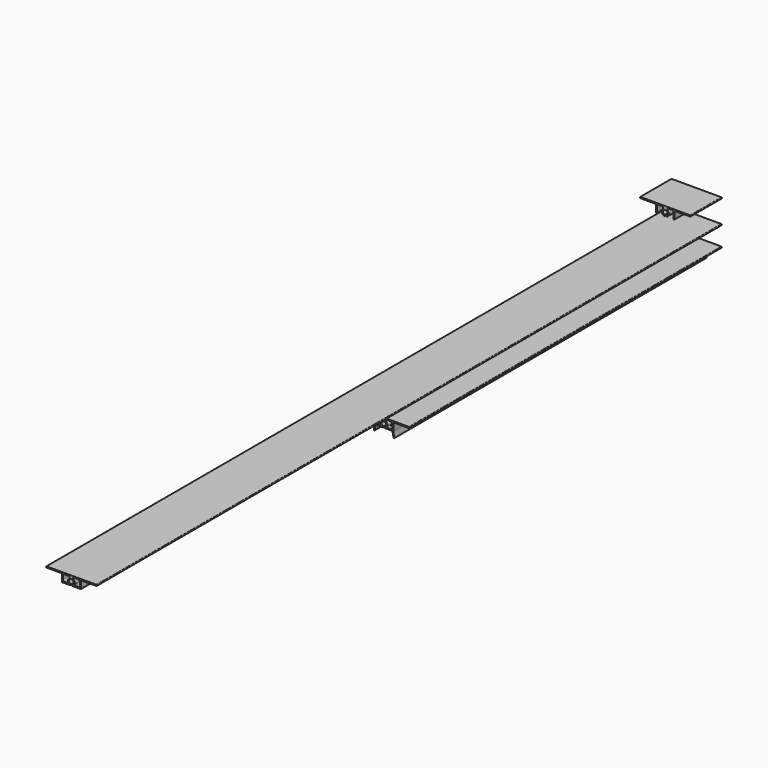
from build123d import *

# Parameters (mm, degrees)
F1_DEPTH = 1000
F2_DEPTH = 2000
F3_DEPTH = 100


# Not quite as in the source:
# - ends of sketch curves that miss each other by under 0.0002 mm in the source are joined


with BuildPart() as f1:
    # F0 (on Front) → F1 (new body)
    with BuildSketch(Plane.XZ):
        with BuildLine():
            Line((63.5, 0), (-63.5, 0))
            ThreePointArc((-63.5, 0), (-65, -1.5), (-63.5, -3))
            Line((-63.5, -3), (-25.2083473523, -3))
            ThreePointArc((-25.2083473523, -3), (-24.5012405711, -3.2928932188), (-24.2083473523, -4))
            Line((-24.2083473523, -4), (-24.2083473523, -22.8776747597))
            ThreePointArc((-24.2083473523, -22.8776747597), (-24.2120777554, -22.9997718388), (-24.223255049, -23.1214134465))
            Line((-24.223255049, -23.1214134465), (-26.0512952001, -38.0096057211))
            ThreePointArc((-26.0512952001, -38.0096057211), (-24.9164089173, -37.5089670967), (-24.2949814984, -36.4354523693))
            Line((-24.2949814984, -36.4354523693), (-21.7759150734, -24.5841766184))
            ThreePointArc((-21.7759150734, -24.5841766184), (-21.0782606541, -23.4457080771), (-19.819619872, -23))
            Line((-19.819619872, -23), (-2.7222222222, -23))
            ThreePointArc((-2.7222222222, -23), (-2.015115441, -22.7071067812), (-1.7222222222, -22))
            Line((-1.7222222222, -22), (-1.7222222222, -20.8607207227))
            ThreePointArc((-1.7222222222, -20.8607207227), (-1.8888888889, -20.3079499243), (-2.3333333333, -19.9394360587))
            ThreePointArc((-2.3333333333, -19.9394360587), (0, -8.4117280748), (2.3333333333, -19.9394360587))
            ThreePointArc((2.3333333333, -19.9394360587), (1.8888888889, -20.3079499243), (1.7222222222, -20.8607207227))
            Line((1.7222222222, -20.8607207227), (1.7222222222, -22))
            ThreePointArc((1.7222222222, -22), (2.015115441, -22.7071067812), (2.7222222222, -23))
            Line((2.7222222222, -23), (19.819619872, -23))
            ThreePointArc((19.819619872, -23), (21.0782606541, -23.4457080771), (21.7759150734, -24.5841766184))
            Line((21.7759150734, -24.5841766184), (24.2949814984, -36.4354523693))
            ThreePointArc((24.2949814984, -36.4354523693), (24.9164089173, -37.5089670967), (26.0512952001, -38.0096057211))
            Line((26.0512952001, -38.0096057211), (24.2381627457, -23.242826893))
            ThreePointArc((24.2381627457, -23.242826893), (24.2269854521, -23.1211852853), (24.223255049, -22.9990882062))
            Line((24.223255049, -22.9990882062), (24.223255049, -3))
            Line((24.223255049, -3), (63.5, -3))
            ThreePointArc((63.5, -3), (65, -1.5), (63.5, 0))
        make_face()
        with BuildLine():
            Line((-21.2083473523, -16), (-21.2083473523, -7))
            ThreePointArc((-21.2083473523, -7), (-20.036774477, -4.1715728753), (-17.2083473523, -3))
            Line((-17.2083473523, -3), (-5.6938014232, -3))
            ThreePointArc((-5.6938014232, -3), (-3.7673478716, -4.4626205124), (-4.6585648008, -6.7112232863))
            ThreePointArc((-4.6585648008, -6.7112232863), (-8.4473321852, -11.3064778509), (-8.5368852816, -17.2615683665))
            ThreePointArc((-8.5368852816, -17.2615683665), (-8.8221800029, -19.1358853065), (-10.5097115925, -20))
            Line((-10.5097115925, -20), (-17.2083473523, -20))
            ThreePointArc((-17.2083473523, -20), (-20.036774477, -18.8284271247), (-21.2083473523, -16))
        make_face(mode=Mode.SUBTRACT)
        with BuildLine():
            Line((21.2083473523, -7), (21.2083473523, -7.008646884))
            Line((21.2083473523, -7.008646884), (21.2083473523, -16))
            ThreePointArc((21.2083473523, -16), (20.036774477, -18.8284271247), (17.2083473523, -20))
            Line((17.2083473523, -20), (10.5097115925, -20))
            ThreePointArc((10.5097115925, -20), (8.8221800029, -19.1358853065), (8.5368852816, -17.2615683665))
            ThreePointArc((8.5368852816, -17.2615683665), (8.4473321852, -11.3064778509), (4.6585648008, -6.7112232863))
            ThreePointArc((4.6585648008, -6.7112232863), (3.7673478716, -4.4626205124), (5.6938014232, -3))
            Line((5.6938014232, -3), (17.2083473523, -3))
            ThreePointArc((17.2083473523, -3), (20.036774477, -4.1715728753), (21.2083473523, -7))
        make_face(mode=Mode.SUBTRACT)
    extrude(amount=F1_DEPTH)


with BuildPart() as f2:
    # F0 (on Front) → F2 (new body)
    with BuildSketch(Plane.XZ):
        with BuildLine():
            Line((63.4000037313, 50.7132201195), (-63.5999962687, 50.7132201195))
            ThreePointArc((-63.5999962687, 50.7132201195), (-65.0999962687, 49.2132201195), (-63.5999962687, 47.7132201195))
            Line((-63.5999962687, 47.7132201195), (-25.308343621, 47.7132201195))
            ThreePointArc((-25.308343621, 47.7132201195), (-24.6012368398, 47.4203269007), (-24.308343621, 46.7132201195))
            Line((-24.308343621, 46.7132201195), (-24.308343621, 28.7132201195))
            ThreePointArc((-24.308343621, 28.7132201195), (-24.0154504022, 28.0061133383), (-23.308343621, 27.7132201195))
            Line((-23.308343621, 27.7132201195), (-19.9187639256, 27.7132201195))
            Line((-19.9187639256, 27.7132201195), (-2.822218491, 27.7132201195))
            ThreePointArc((-2.822218491, 27.7132201195), (-2.1151117098, 28.0061133383), (-1.822218491, 28.7132201195))
            Line((-1.822218491, 28.7132201195), (-1.822218491, 29.8524993968))
            ThreePointArc((-1.822218491, 29.8524993968), (-1.9888851576, 30.4052701952), (-2.4333296021, 30.7737840608))
            ThreePointArc((-2.4333296021, 30.7737840608), (-0.0999962687, 42.3014920447), (2.2333370646, 30.7737840608))
            ThreePointArc((2.2333370646, 30.7737840608), (1.7888926201, 30.4052701952), (1.6222259535, 29.8524993968))
            Line((1.6222259535, 29.8524993968), (1.6222259535, 28.7132201195))
            ThreePointArc((1.6222259535, 28.7132201195), (1.9151191723, 28.0061133383), (2.6222259535, 27.7132201195))
            Line((2.6222259535, 27.7132201195), (19.7196236032, 27.7132201195))
            Line((19.7196236032, 27.7132201195), (23.629926187, 27.7132201195))
            ThreePointArc((23.629926187, 27.7132201195), (24.3370329682, 28.0061133383), (24.629926187, 28.7132201195))
            Line((24.629926187, 28.7132201195), (24.629926187, 47.7132201195))
            Line((24.629926187, 47.7132201195), (63.4000037313, 47.7132201195))
            ThreePointArc((63.4000037313, 47.7132201195), (64.9000037313, 49.2132201195), (63.4000037313, 50.7132201195))
        make_face()
        with BuildLine():
            Line((-21.308343621, 34.7132201195), (-21.308343621, 43.7132201195))
            ThreePointArc((-21.308343621, 43.7132201195), (-20.1367707458, 46.5416472442), (-17.308343621, 47.7132201195))
            Line((-17.308343621, 47.7132201195), (-5.7937976919, 47.7132201195))
            ThreePointArc((-5.7937976919, 47.7132201195), (-3.8673441404, 46.2505996071), (-4.7585610695, 44.0019968332))
            ThreePointArc((-4.7585610695, 44.0019968332), (-8.5473284539, 39.4067422686), (-8.6368815504, 33.451651753))
            ThreePointArc((-8.6368815504, 33.451651753), (-8.9221762716, 31.577334813), (-10.6097078613, 30.7132201195))
            Line((-10.6097078613, 30.7132201195), (-17.308343621, 30.7132201195))
            ThreePointArc((-17.308343621, 30.7132201195), (-20.1367707458, 31.8847929947), (-21.308343621, 34.7132201195))
        make_face(mode=Mode.SUBTRACT)
        with BuildLine():
            Line((21.629926187, 43.7218670034), (21.629926187, 43.7132201195))
            Line((21.629926187, 43.7132201195), (21.629926187, 34.7132201195))
            ThreePointArc((21.629926187, 34.7132201195), (20.4583533118, 31.8847929947), (17.629926187, 30.7132201195))
            Line((17.629926187, 30.7132201195), (17.1083510835, 30.7132201195))
            Line((17.1083510835, 30.7132201195), (10.4097153238, 30.7132201195))
            ThreePointArc((10.4097153238, 30.7132201195), (8.7221837341, 31.577334813), (8.4368890129, 33.451651753))
            ThreePointArc((8.4368890129, 33.451651753), (8.3473359164, 39.4067422686), (4.558568532, 44.0019968332))
            ThreePointArc((4.558568532, 44.0019968332), (3.6673516029, 46.2505996071), (5.5938051544, 47.7132201195))
            Line((5.5938051544, 47.7132201195), (6.115380258, 47.7132201195))
            Line((6.115380258, 47.7132201195), (17.629926187, 47.7132201195))
            ThreePointArc((17.629926187, 47.7132201195), (20.4552945298, 46.5447027218), (21.629926187, 43.7218670034))
        make_face(mode=Mode.SUBTRACT)
    extrude(amount=F2_DEPTH)


with BuildPart() as f3:
    # F0 (on Front) → F3 (new body)
    with BuildSketch(Plane.XZ):
        with BuildLine():
            Line((63.6676191584, 111.000010252), (-63.3110105991, 111.000010252))
            ThreePointArc((-63.3110105991, 111.000010252), (-64.8110105991, 109.500010252), (-63.3110105991, 108.000010252))
            Line((-63.3110105991, 108.000010252), (-25.0193579514, 108.000010252))
            ThreePointArc((-25.0193579514, 108.000010252), (-24.3122511702, 107.7071170332), (-24.0193579514, 107.000010252))
            Line((-24.0193579514, 107.000010252), (-24.0193579514, 89.4322879863))
            ThreePointArc((-24.0193579514, 89.4322879863), (-23.5800181232, 88.3716278145), (-22.5193579514, 87.9322879863))
            ThreePointArc((-22.5193579514, 87.9322879863), (-21.4586977796, 88.3716278145), (-21.0193579514, 89.4322879863))
            Line((-21.0193579514, 89.4322879863), (-21.0193579514, 104.000010252))
            ThreePointArc((-21.0193579514, 104.000010252), (-19.8477850761, 106.8284373767), (-17.0193579514, 108.000010252))
            Line((-17.0193579514, 108.000010252), (-8.2922328934, 108.000010252))
            ThreePointArc((-8.2922328934, 108.000010252), (-5.5195987668, 106.1456541757), (-6.1745986001, 102.875010252))
            ThreePointArc((-6.1745986001, 102.875010252), (-8.5862177235, 94.4547342177), (-2.6967573079, 87.9715859621))
            ThreePointArc((-2.6967573079, 87.9715859621), (-2.4524791129, 87.9323026488), (-2.2087112857, 87.9746377601))
            ThreePointArc((-2.2087112857, 87.9746377601), (-1.7241213898, 88.3399312814), (-1.5399880278, 88.918171395))
            Line((-1.5399880278, 88.918171395), (-1.5399880278, 90.0404468849))
            ThreePointArc((-1.5399880278, 90.0404468849), (-1.6723445466, 90.5376337608), (-2.0343776068, 90.9032087885))
            ThreePointArc((-2.0343776068, 90.9032087885), (0.1783042796, 102.4803082917), (2.3909861661, 90.9032087885))
            ThreePointArc((2.3909861661, 90.9032087885), (2.0289531059, 90.5376337608), (1.8965965871, 90.0404468849))
            Line((1.8965965871, 90.0404468849), (1.8965965871, 88.918171395))
            ThreePointArc((1.8965965871, 88.918171395), (2.080729949, 88.3399312814), (2.565319845, 87.9746377601))
            ThreePointArc((2.565319845, 87.9746377601), (2.8090876722, 87.9323026488), (3.0533658672, 87.9715859621))
            ThreePointArc((3.0533658672, 87.9715859621), (8.9428262828, 94.4547342177), (6.5312071594, 102.875010252))
            ThreePointArc((6.5312071594, 102.875010252), (5.8762073261, 106.1456541757), (8.6488414527, 108.000010252))
            Line((8.6488414527, 108.000010252), (17.3759665107, 108.000010252))
            ThreePointArc((17.3759665107, 108.000010252), (20.2043936354, 106.8284373767), (21.3759665107, 104.000010252))
            Line((21.3759665107, 104.000010252), (21.3759665107, 89.4322879863))
            ThreePointArc((21.3759665107, 89.4322879863), (21.8153063389, 88.3716278145), (22.8759665107, 87.9322879863))
            ThreePointArc((22.8759665107, 87.9322879863), (23.9366266825, 88.3716278145), (24.3759665107, 89.4322879863))
            Line((24.3759665107, 89.4322879863), (24.3759665107, 107.000010252))
            ThreePointArc((24.3759665107, 107.000010252), (24.6688597295, 107.7071170332), (25.3759665107, 108.000010252))
            Line((25.3759665107, 108.000010252), (63.6676191584, 108.000010252))
            ThreePointArc((63.6676191584, 108.000010252), (65.1676191584, 109.500010252), (63.6676191584, 111.000010252))
        make_face()
    extrude(amount=F3_DEPTH)


solid = Compound([f1.part, f2.part, f3.part])
